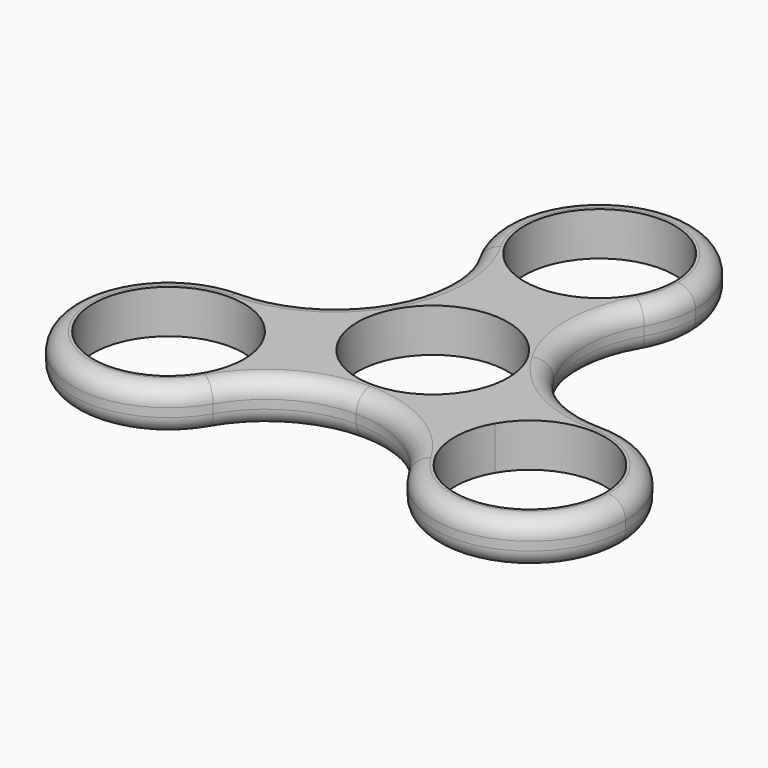
from build123d import *

# Parameters (mm, degrees)
F0_R     = 10.9982
F1_DEPTH = 6.35
F2_R     = 2.54
F3_R     = 2.54


with BuildPart() as f1:
    # F0 (on Top) → F1 (new body)
    with BuildSketch(Plane.XY):
        with BuildLine():
            ThreePointArc((9.5247205959, 5.4991), (10.6234454227, 2.8465436218), (10.9982, 0))
            ThreePointArc((10.9982, 0), (10.6234454227, -2.8465436218), (9.5247205959, -5.4991))
            Line((9.5247205959, -5.4991), (12.0983748909, -6.985))
            ThreePointArc((12.0983748909, -6.985), (13.4939837933, -3.6157020601), (13.97, 0))
            ThreePointArc((13.97, 0), (13.4939837933, 3.6157020601), (12.0983748909, 6.985))
            Line((12.0983748909, 6.985), (9.5247205959, 5.4991))
        make_face()
        with BuildLine():
            ThreePointArc((0, 10.9982), (5.4991, 9.5247205959), (9.5247205959, 5.4991))
            Line((9.5247205959, 5.4991), (12.0983748909, 6.985))
            ThreePointArc((12.0983748909, 6.985), (6.985, 12.0983748909), (0, 13.97))
            Line((0, 13.97), (0, 10.9982))
        make_face()
        with BuildLine():
            Line((12.0983748909, -6.985), (9.5247205959, -5.4991))
            ThreePointArc((9.5247205959, -5.4991), (-9.5247205959, -5.4991), (0, 10.9982))
            Line((0, 10.9982), (0, 13.97))
            ThreePointArc((0, 13.97), (-6.985, 12.0983748909), (-12.0983748909, 6.985))
            ThreePointArc((-12.0983748909, 6.985), (-12.0983748909, -6.985), (0, -13.97))
            ThreePointArc((0, -13.97), (6.985, -12.0983748909), (12.0983748909, -6.985))
        make_face()
        with BuildLine():
            ThreePointArc((26.3964543073, -1.27), (18.1414543073, 0.9419205835), (12.0983748909, 6.985))
            ThreePointArc((12.0983748909, 6.985), (13.4939837933, 3.6157020601), (13.97, 0))
            ThreePointArc((13.97, 0), (13.4939837933, -3.6157020601), (12.0983748909, -6.985))
            Line((12.0983748909, -6.985), (14.2980794165, -8.255))
            ThreePointArc((14.2980794165, -8.255), (19.4114543073, -3.1416251091), (26.3964543073, -1.27))
        make_face()
        with BuildLine():
            ThreePointArc((0, 13.97), (6.985, 12.0983748909), (12.0983748909, 6.985))
            ThreePointArc((12.0983748909, 6.985), (9.8864543073, 15.24), (12.0983748909, 23.495))
            ThreePointArc((12.0983748909, 23.495), (6.985, 18.3816251091), (0, 16.51))
            Line((0, 16.51), (0, 13.97))
        make_face()
        with BuildLine():
            Line((14.2980794165, -8.255), (12.0983748909, -6.985))
            ThreePointArc((12.0983748909, -6.985), (6.985, -12.0983748909), (0, -13.97))
            ThreePointArc((0, -13.97), (8.255, -16.1819205835), (14.2980794165, -22.225))
            ThreePointArc((14.2980794165, -22.225), (12.4264543073, -15.24), (14.2980794165, -8.255))
        make_face()
        with BuildLine():
            ThreePointArc((-12.0983748909, 6.985), (-6.985, 12.0983748909), (0, 13.97))
            Line((0, 13.97), (0, 16.51))
            ThreePointArc((0, 16.51), (-6.985, 18.3816251091), (-12.0983748909, 23.495))
            ThreePointArc((-12.0983748909, 23.495), (-9.8864543073, 15.24), (-12.0983748909, 6.985))
        make_face()
        with BuildLine():
            ThreePointArc((0, 16.51), (6.985, 18.3816251091), (12.0983748909, 23.495))
            ThreePointArc((12.0983748909, 23.495), (13.4939837933, 26.8642979399), (13.97, 30.48))
            ThreePointArc((13.97, 30.48), (-3.6157020601, 43.9739837933), (-12.0983748909, 23.495))
            ThreePointArc((-12.0983748909, 23.495), (-6.985, 18.3816251091), (0, 16.51))
        make_face()
        with BuildLine():
            ThreePointArc((10.9982, 30.48), (7.7769018008, 22.7030981992), (0, 19.4818))
            ThreePointArc((0, 19.4818), (-7.7769018008, 38.2569018008), (10.9982, 30.48))
        make_face(mode=Mode.SUBTRACT)
        with BuildLine():
            ThreePointArc((40.3664543073, -15.24), (36.2747360405, -5.3617182668), (26.3964543073, -1.27))
            ThreePointArc((26.3964543073, -1.27), (19.4114543073, -3.1416251091), (14.2980794165, -8.255))
            ThreePointArc((14.2980794165, -8.255), (12.4264543073, -15.24), (14.2980794165, -22.225))
            ThreePointArc((14.2980794165, -22.225), (30.0121563674, -28.7339837933), (40.3664543073, -15.24))
        make_face()
        with BuildLine():
            ThreePointArc((37.3946543073, -15.24), (23.5499106855, -25.8634454227), (16.8717337114, -9.7409))
            ThreePointArc((16.8717337114, -9.7409), (29.2429979292, -4.6165545773), (37.3946543073, -15.24))
        make_face(mode=Mode.SUBTRACT)
        with BuildLine():
            ThreePointArc((-14.2980794165, -22.225), (-8.255, -16.1819205835), (0, -13.97))
            ThreePointArc((0, -13.97), (-12.0983748909, -6.985), (-12.0983748909, 6.985))
            ThreePointArc((-12.0983748909, 6.985), (-18.1414543073, 0.9419205835), (-26.3964543073, -1.27))
            ThreePointArc((-26.3964543073, -1.27), (-16.5181725742, -5.3617182668), (-12.4264543073, -15.24))
            ThreePointArc((-12.4264543073, -15.24), (-12.9024705141, -18.8557020601), (-14.2980794165, -22.225))
        make_face()
        with BuildLine():
            ThreePointArc((-26.3964543073, -1.27), (-38.4948291982, -22.225), (-14.2980794165, -22.225))
            ThreePointArc((-14.2980794165, -22.225), (-12.9024705141, -18.8557020601), (-12.4264543073, -15.24))
            ThreePointArc((-12.4264543073, -15.24), (-16.5181725742, -5.3617182668), (-26.3964543073, -1.27))
        make_face()
        with Locations((-26.3964543073, -15.24)):
            Circle(F0_R, mode=Mode.SUBTRACT)
    extrude(amount=F1_DEPTH)

    # F2
    f2_edges = [f1.edges().sort_by_distance(p)[0] for p in [
        (-38.494829, -22.225, 6.35),
        (0, -13.97, 6.35),
        (38.494829, -22.225, 6.35),
        (0, 44.45, 6.35),
        (12.098375, 6.985, 6.35),
        (-12.098375, 6.985, 6.35),
    ]]
    fillet(f2_edges, radius=F2_R)

    # F3
    f3_edges = [f1.edges().sort_by_distance(p)[0] for p in [
        (38.494829, -22.225, 0),
        (12.098375, 6.985, 0),
        (0, 44.45, 0),
        (-12.098375, 6.985, 0),
        (-38.494829, -22.225, 0),
        (0, -13.97, 0),
    ]]
    fillet(f3_edges, radius=F3_R)


solid = f1.part
